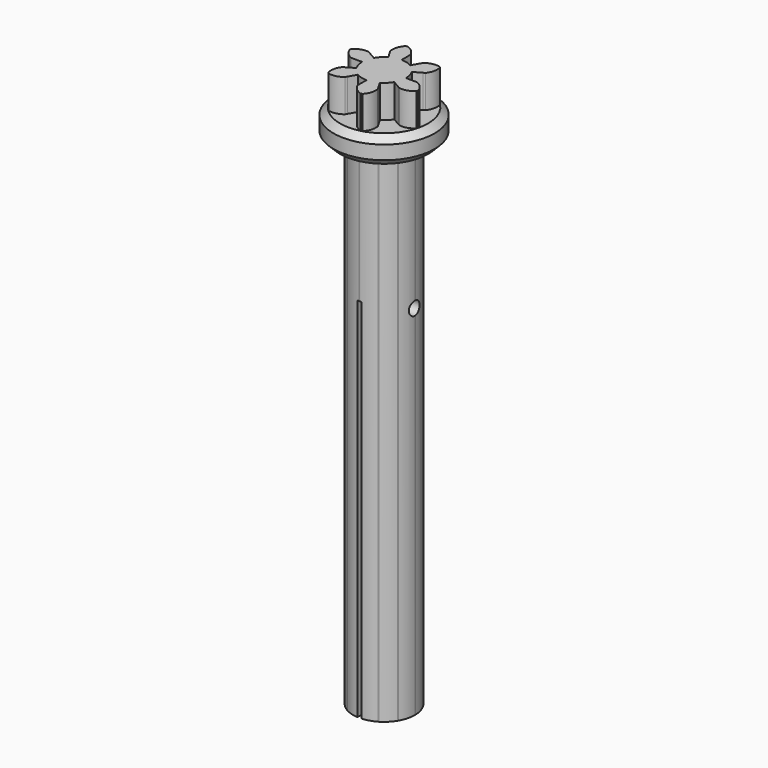
from build123d import *

# Parameters (mm, degrees)
F6_DEPTH       = 5
F7_DEPTH       = 80
F9_START       = -75.9
F8_R           = 7.6984631039
F9_DEPTH       = 4.1
F10_SIZE       = 1
F11_DEPTH      = 55.9
F12_R          = 1.025
F13_DEPTH      = 7.6994631039
F13_DEPTH_BACK = 7.6994631039


# Not quite as in the source:
# - a feature names something its author has since deleted; it is built from what else it names


with BuildPart() as f6:
    # F5 (on Top) → F6 (new body)
    with BuildSketch(Plane.XY):
        with BuildLine():
            Line((-4.0689884067, 2.349231552), (-4.3301270189, 2.5))
            ThreePointArc((-4.3301270189, 2.5), (-4.8296291314, 1.2940952255), (-5, 0))
            Line((-5, 0), (-4.6984631039, 0))
            ThreePointArc((-4.6984631039, 0), (-4.538366856, 1.216051734), (-4.0689884067, 2.349231552))
        make_face()
        with BuildLine():
            Line((-2.8867513459, 1.6666666667), (-4.0689884067, 2.349231552))
            ThreePointArc((-4.0689884067, 2.349231552), (-4.538366856, 1.216051734), (-4.6984631039, 0))
            Line((-4.6984631039, 0), (-3.3333333333, 0))
            ThreePointArc((-3.3333333333, 0), (-3.2197527543, 0.8627301503), (-2.8867513459, 1.6666666667))
        make_face()
        with BuildLine():
            ThreePointArc((-2.5, 4.3301270189), (-1.2940952255, 4.8296291314), (0, 5))
            ThreePointArc((0, 5), (-0.6289197853, 5.9186828799), (-1.5943250641, 6.4732196035))
            Line((-1.5943250641, 6.4732196035), (-1.7258162456, 6.440833913))
            Line((-1.7258162456, 6.440833913), (-1.8558837944, 6.4031351529))
            ThreePointArc((-1.8558837944, 6.4031351529), (-2.414680929, 5.4401896236), (-2.5, 4.3301270189))
        make_face()
        with BuildLine():
            ThreePointArc((2.8867513459, -1.6666666667), (3.2197527543, -0.8627301503), (3.3333333333, 0))
            ThreePointArc((3.3333333333, 0), (3.2197527543, 0.8627301503), (2.8867513459, 1.6666666667))
            ThreePointArc((2.8867513459, 1.6666666667), (2.357022604, 2.357022604), (1.6666666667, 2.8867513459))
            ThreePointArc((1.6666666667, 2.8867513459), (0.8627301503, 3.2197527543), (0, 3.3333333333))
            ThreePointArc((0, 3.3333333333), (-0.8627301503, 3.2197527543), (-1.6666666667, 2.8867513459))
            ThreePointArc((-1.6666666667, 2.8867513459), (-2.357022604, 2.357022604), (-2.8867513459, 1.6666666667))
            ThreePointArc((-2.8867513459, 1.6666666667), (-3.2197527543, 0.8627301503), (-3.3333333333, 0))
            ThreePointArc((-3.3333333333, 0), (-3.2197527543, -0.8627301503), (-2.8867513459, -1.6666666667))
            ThreePointArc((-2.8867513459, -1.6666666667), (-2.357022604, -2.357022604), (-1.6666666667, -2.8867513459))
            ThreePointArc((-1.6666666667, -2.8867513459), (-0.8627301503, -3.2197527543), (0, -3.3333333333))
            ThreePointArc((0, -3.3333333333), (0.8627301503, -3.2197527543), (1.6666666667, -2.8867513459))
            ThreePointArc((1.6666666667, -2.8867513459), (2.357022604, -2.357022604), (2.8867513459, -1.6666666667))
        make_face()
        with BuildLine():
            Line((4.0689884067, 2.349231552), (4.3301270189, 2.5))
            ThreePointArc((4.3301270189, 2.5), (3.5355339059, 3.5355339059), (2.5, 4.3301270189))
            Line((2.5, 4.3301270189), (2.349231552, 4.0689884067))
            ThreePointArc((2.349231552, 4.0689884067), (3.3223151219, 3.3223151219), (4.0689884067, 2.349231552))
        make_face()
        with BuildLine():
            Line((2.8867513459, 1.6666666667), (4.0689884067, 2.349231552))
            ThreePointArc((4.0689884067, 2.349231552), (3.3223151219, 3.3223151219), (2.349231552, 4.0689884067))
            Line((2.349231552, 4.0689884067), (1.6666666667, 2.8867513459))
            ThreePointArc((1.6666666667, 2.8867513459), (2.357022604, 2.357022604), (2.8867513459, 1.6666666667))
        make_face()
        with BuildLine():
            ThreePointArc((4.3301270189, -2.5), (4.8296291314, -1.2940952255), (5, 0))
            Line((5, 0), (4.6984631039, 0))
            ThreePointArc((4.6984631039, 0), (4.538366856, -1.216051734), (4.0689884067, -2.349231552))
            Line((4.0689884067, -2.349231552), (4.3301270189, -2.5))
        make_face()
        with BuildLine():
            ThreePointArc((4.0689884067, -2.349231552), (4.538366856, -1.216051734), (4.6984631039, 0))
            Line((4.6984631039, 0), (3.3333333333, 0))
            ThreePointArc((3.3333333333, 0), (3.2197527543, -0.8627301503), (2.8867513459, -1.6666666667))
            Line((2.8867513459, -1.6666666667), (4.0689884067, -2.349231552))
        make_face()
        with BuildLine():
            ThreePointArc((0, -5), (1.2940952255, -4.8296291314), (2.5, -4.3301270189))
            Line((2.5, -4.3301270189), (2.349231552, -4.0689884067))
            ThreePointArc((2.349231552, -4.0689884067), (1.216051734, -4.538366856), (0, -4.6984631039))
            Line((0, -4.6984631039), (0, -5))
        make_face()
        with BuildLine():
            ThreePointArc((0, -4.6984631039), (1.216051734, -4.538366856), (2.349231552, -4.0689884067))
            Line((2.349231552, -4.0689884067), (1.6666666667, -2.8867513459))
            ThreePointArc((1.6666666667, -2.8867513459), (0.8627301503, -3.2197527543), (0, -3.3333333333))
            Line((0, -3.3333333333), (0, -4.6984631039))
        make_face()
        with BuildLine():
            ThreePointArc((-4.3301270189, -2.5), (-3.5355339059, -3.5355339059), (-2.5, -4.3301270189))
            Line((-2.5, -4.3301270189), (-2.349231552, -4.0689884067))
            ThreePointArc((-2.349231552, -4.0689884067), (-3.3223151219, -3.3223151219), (-4.0689884067, -2.349231552))
            Line((-4.0689884067, -2.349231552), (-4.3301270189, -2.5))
        make_face()
        with BuildLine():
            ThreePointArc((-4.0689884067, -2.349231552), (-3.3223151219, -3.3223151219), (-2.349231552, -4.0689884067))
            Line((-2.349231552, -4.0689884067), (-1.6666666667, -2.8867513459))
            ThreePointArc((-1.6666666667, -2.8867513459), (-2.357022604, -2.357022604), (-2.8867513459, -1.6666666667))
            Line((-2.8867513459, -1.6666666667), (-4.0689884067, -2.349231552))
        make_face()
        with BuildLine():
            Line((0, 4.6984631039), (0, 5))
            ThreePointArc((0, 5), (-1.2940952255, 4.8296291314), (-2.5, 4.3301270189))
            Line((-2.5, 4.3301270189), (-2.349231552, 4.0689884067))
            ThreePointArc((-2.349231552, 4.0689884067), (-1.216051734, 4.538366856), (0, 4.6984631039))
        make_face()
        with BuildLine():
            Line((0, 3.3333333333), (0, 4.6984631039))
            ThreePointArc((0, 4.6984631039), (-1.216051734, 4.538366856), (-2.349231552, 4.0689884067))
            Line((-2.349231552, 4.0689884067), (-1.6666666667, 2.8867513459))
            ThreePointArc((-1.6666666667, 2.8867513459), (-0.8627301503, 3.2197527543), (0, 3.3333333333))
        make_face()
        with BuildLine():
            ThreePointArc((-5, 0), (-4.8296291314, 1.2940952255), (-4.3301270189, 2.5))
            ThreePointArc((-4.3301270189, 2.5), (-5.4401896236, 2.414680929), (-6.4031351529, 1.8558837944))
            Line((-6.4031351529, 1.8558837944), (-6.440833913, 1.7258162456))
            Line((-6.440833913, 1.7258162456), (-6.4732196035, 1.5943250641))
            ThreePointArc((-6.4732196035, 1.5943250641), (-5.9186828799, 0.6289197853), (-5, 0))
        make_face()
        with BuildLine():
            ThreePointArc((-4.6173358091, -4.8088100888), (-3.5040019509, -4.8112698383), (-2.5, -4.3301270189))
            ThreePointArc((-2.5, -4.3301270189), (-3.5355339059, -3.5355339059), (-4.3301270189, -2.5))
            ThreePointArc((-4.3301270189, -2.5), (-4.8112698383, -3.5040019509), (-4.8088100888, -4.6173358091))
            Line((-4.8088100888, -4.6173358091), (-4.7150176674, -4.7150176674))
            Line((-4.7150176674, -4.7150176674), (-4.6173358091, -4.8088100888))
        make_face()
        with BuildLine():
            ThreePointArc((1.8558837944, -6.4031351529), (2.414680929, -5.4401896236), (2.5, -4.3301270189))
            ThreePointArc((2.5, -4.3301270189), (1.2940952255, -4.8296291314), (0, -5))
            ThreePointArc((0, -5), (0.6289197853, -5.9186828799), (1.5943250641, -6.4732196035))
            Line((1.5943250641, -6.4732196035), (1.7258162456, -6.440833913))
            Line((1.7258162456, -6.440833913), (1.8558837944, -6.4031351529))
        make_face()
        with BuildLine():
            ThreePointArc((6.4732196035, -1.5943250641), (5.9186828799, -0.6289197853), (5, 0))
            ThreePointArc((5, 0), (4.8296291314, -1.2940952255), (4.3301270189, -2.5))
            ThreePointArc((4.3301270189, -2.5), (5.4401896236, -2.414680929), (6.4031351529, -1.8558837944))
            Line((6.4031351529, -1.8558837944), (6.440833913, -1.7258162456))
            Line((6.440833913, -1.7258162456), (6.4732196035, -1.5943250641))
        make_face()
        with BuildLine():
            ThreePointArc((2.5, 4.3301270189), (3.5355339059, 3.5355339059), (4.3301270189, 2.5))
            ThreePointArc((4.3301270189, 2.5), (4.8112698383, 3.5040019509), (4.8088100888, 4.6173358091))
            Line((4.8088100888, 4.6173358091), (4.7150176674, 4.7150176674))
            Line((4.7150176674, 4.7150176674), (4.6173358091, 4.8088100888))
            ThreePointArc((4.6173358091, 4.8088100888), (3.5040019509, 4.8112698383), (2.5, 4.3301270189))
        make_face()
    extrude(amount=F6_DEPTH)

    # F5 (on Top) → F7 (join)
    with BuildSketch(Plane.XY):
        with BuildLine():
            ThreePointArc((2.8867513459, -1.6666666667), (3.2197527543, -0.8627301503), (3.3333333333, 0))
            ThreePointArc((3.3333333333, 0), (3.2197527543, 0.8627301503), (2.8867513459, 1.6666666667))
            ThreePointArc((2.8867513459, 1.6666666667), (2.357022604, 2.357022604), (1.6666666667, 2.8867513459))
            ThreePointArc((1.6666666667, 2.8867513459), (0.8627301503, 3.2197527543), (0, 3.3333333333))
            ThreePointArc((0, 3.3333333333), (-0.8627301503, 3.2197527543), (-1.6666666667, 2.8867513459))
            ThreePointArc((-1.6666666667, 2.8867513459), (-2.357022604, 2.357022604), (-2.8867513459, 1.6666666667))
            ThreePointArc((-2.8867513459, 1.6666666667), (-3.2197527543, 0.8627301503), (-3.3333333333, 0))
            ThreePointArc((-3.3333333333, 0), (-3.2197527543, -0.8627301503), (-2.8867513459, -1.6666666667))
            ThreePointArc((-2.8867513459, -1.6666666667), (-2.357022604, -2.357022604), (-1.6666666667, -2.8867513459))
            ThreePointArc((-1.6666666667, -2.8867513459), (-0.8627301503, -3.2197527543), (0, -3.3333333333))
            ThreePointArc((0, -3.3333333333), (0.8627301503, -3.2197527543), (1.6666666667, -2.8867513459))
            ThreePointArc((1.6666666667, -2.8867513459), (2.357022604, -2.357022604), (2.8867513459, -1.6666666667))
        make_face()
        with BuildLine():
            ThreePointArc((-4.1169236265, -2.2641765374), (-4.0931769499, -2.306828558), (-4.0689884067, -2.349231552))
            Line((-4.0689884067, -2.349231552), (-2.8867513459, -1.6666666667))
            ThreePointArc((-2.8867513459, -1.6666666667), (-3.2197527543, -0.8627301503), (-3.3333333333, 0))
            Line((-3.3333333333, 0), (-4.6984631039, 0))
            ThreePointArc((-4.6984631039, 0), (-4.6982094998, -0.0488163415), (-4.6974487147, -0.0976274132))
            ThreePointArc((-4.6974487147, -0.0976274132), (-4.538366856, -1.216051734), (-4.1169236265, -2.2641765374))
        make_face()
        with BuildLine():
            Line((-2.8867513459, 1.6666666667), (-4.0689884067, 2.349231552))
            ThreePointArc((-4.0689884067, 2.349231552), (-4.538366856, 1.216051734), (-4.6984631039, 0))
            Line((-4.6984631039, 0), (-3.3333333333, 0))
            ThreePointArc((-3.3333333333, 0), (-3.2197527543, 0.8627301503), (-2.8867513459, 1.6666666667))
        make_face()
        with BuildLine():
            ThreePointArc((-2.349231552, 4.0689884067), (-2.3913809418, 4.0443606083), (-2.4332721773, 4.0192962133))
            ThreePointArc((-2.4332721773, 4.0192962133), (-3.3223151219, 3.3223151219), (-4.0192962133, 2.4332721773))
            ThreePointArc((-4.0192962133, 2.4332721773), (-4.0443606083, 2.3913809418), (-4.0689884067, 2.349231552))
            Line((-4.0689884067, 2.349231552), (-2.8867513459, 1.6666666667))
            ThreePointArc((-2.8867513459, 1.6666666667), (-2.357022604, 2.357022604), (-1.6666666667, 2.8867513459))
            Line((-1.6666666667, 2.8867513459), (-2.349231552, 4.0689884067))
        make_face()
        with BuildLine():
            Line((0, 3.3333333333), (0, 4.6984631039))
            ThreePointArc((0, 4.6984631039), (-1.216051734, 4.538366856), (-2.349231552, 4.0689884067))
            Line((-2.349231552, 4.0689884067), (-1.6666666667, 2.8867513459))
            ThreePointArc((-1.6666666667, 2.8867513459), (-0.8627301503, 3.2197527543), (0, 3.3333333333))
        make_face()
        with BuildLine():
            ThreePointArc((2.349231552, 4.0689884067), (2.306828558, 4.0931769499), (2.2641765374, 4.1169236265))
            ThreePointArc((2.2641765374, 4.1169236265), (1.216051734, 4.538366856), (0.0976274132, 4.6974487147))
            ThreePointArc((0.0976274132, 4.6974487147), (0.0488163415, 4.6982094998), (0, 4.6984631039))
            Line((0, 4.6984631039), (0, 3.3333333333))
            ThreePointArc((0, 3.3333333333), (0.8627301503, 3.2197527543), (1.6666666667, 2.8867513459))
            Line((1.6666666667, 2.8867513459), (2.349231552, 4.0689884067))
        make_face()
        with BuildLine():
            Line((2.8867513459, 1.6666666667), (4.0689884067, 2.349231552))
            ThreePointArc((4.0689884067, 2.349231552), (3.3223151219, 3.3223151219), (2.349231552, 4.0689884067))
            Line((2.349231552, 4.0689884067), (1.6666666667, 2.8867513459))
            ThreePointArc((1.6666666667, 2.8867513459), (2.357022604, 2.357022604), (2.8867513459, 1.6666666667))
        make_face()
        with BuildLine():
            ThreePointArc((4.6984631039, 0), (4.6982094998, 0.0488163415), (4.6974487147, 0.0976274132))
            ThreePointArc((4.6974487147, 0.0976274132), (4.538366856, 1.216051734), (4.1169236265, 2.2641765374))
            ThreePointArc((4.1169236265, 2.2641765374), (4.0931769499, 2.306828558), (4.0689884067, 2.349231552))
            Line((4.0689884067, 2.349231552), (2.8867513459, 1.6666666667))
            ThreePointArc((2.8867513459, 1.6666666667), (3.2197527543, 0.8627301503), (3.3333333333, 0))
            Line((3.3333333333, 0), (4.6984631039, 0))
        make_face()
        with BuildLine():
            ThreePointArc((4.0689884067, -2.349231552), (4.538366856, -1.216051734), (4.6984631039, 0))
            Line((4.6984631039, 0), (3.3333333333, 0))
            ThreePointArc((3.3333333333, 0), (3.2197527543, -0.8627301503), (2.8867513459, -1.6666666667))
            Line((2.8867513459, -1.6666666667), (4.0689884067, -2.349231552))
        make_face()
        with BuildLine():
            ThreePointArc((4.0192962133, -2.4332721773), (4.0443606083, -2.3913809418), (4.0689884067, -2.349231552))
            Line((4.0689884067, -2.349231552), (2.8867513459, -1.6666666667))
            ThreePointArc((2.8867513459, -1.6666666667), (2.357022604, -2.357022604), (1.6666666667, -2.8867513459))
            Line((1.6666666667, -2.8867513459), (2.349231552, -4.0689884067))
            ThreePointArc((2.349231552, -4.0689884067), (2.3913809418, -4.0443606083), (2.4332721773, -4.0192962133))
            ThreePointArc((2.4332721773, -4.0192962133), (3.3223151219, -3.3223151219), (4.0192962133, -2.4332721773))
        make_face()
        with BuildLine():
            ThreePointArc((0, -4.6984631039), (1.216051734, -4.538366856), (2.349231552, -4.0689884067))
            Line((2.349231552, -4.0689884067), (1.6666666667, -2.8867513459))
            ThreePointArc((1.6666666667, -2.8867513459), (0.8627301503, -3.2197527543), (0, -3.3333333333))
            Line((0, -3.3333333333), (0, -4.6984631039))
        make_face()
        with BuildLine():
            ThreePointArc((-0.0976274132, -4.6974487147), (-0.0488163415, -4.6982094998), (0, -4.6984631039))
            Line((0, -4.6984631039), (0, -3.3333333333))
            ThreePointArc((0, -3.3333333333), (-0.8627301503, -3.2197527543), (-1.6666666667, -2.8867513459))
            Line((-1.6666666667, -2.8867513459), (-2.349231552, -4.0689884067))
            ThreePointArc((-2.349231552, -4.0689884067), (-2.306828558, -4.0931769499), (-2.2641765374, -4.1169236265))
            ThreePointArc((-2.2641765374, -4.1169236265), (-1.216051734, -4.538366856), (-0.0976274132, -4.6974487147))
        make_face()
        with BuildLine():
            ThreePointArc((-4.0689884067, -2.349231552), (-3.3223151219, -3.3223151219), (-2.349231552, -4.0689884067))
            Line((-2.349231552, -4.0689884067), (-1.6666666667, -2.8867513459))
            ThreePointArc((-1.6666666667, -2.8867513459), (-2.357022604, -2.357022604), (-2.8867513459, -1.6666666667))
            Line((-2.8867513459, -1.6666666667), (-4.0689884067, -2.349231552))
        make_face()
    extrude(amount=-F7_DEPTH)

    # F8 (on face) → F9 (join)
    with BuildSketch(Plane(origin=(0, 0, -80), x_dir=(1, 0, 0), z_dir=(0, 0, -1)).offset(F9_START)):
        Circle(F8_R)
        with BuildLine():
            ThreePointArc((-0.3, -4.6888757223), (-4.6984631039, 0), (-0.3, 4.6888757223))
            ThreePointArc((-0.3, 4.6888757223), (0, 4.6984631039), (0.3, 4.6888757223))
            ThreePointArc((0.3, 4.6888757223), (3.4267400303, 3.2144996973), (4.6984631039, 0))
            ThreePointArc((4.6984631039, 0), (3.4267400303, -3.2144996973), (0.3, -4.6888757223))
            ThreePointArc((0.3, -4.6888757223), (0, -4.6984631039), (-0.3, -4.6888757223))
        make_face(mode=Mode.SUBTRACT)
    extrude(amount=-F9_DEPTH)

    # F10
    f10_edges = [f6.edges().sort_by_distance(p)[0] for p in [
        (-7.698463, 0, 0),
        (-7.698463, 0, -4.1),
    ]]
    chamfer(f10_edges, length=F10_SIZE)

    # F8 (on face) → F11 (cut)
    with BuildSketch(Plane(origin=(0, 0, -80), x_dir=(1, 0, 0), z_dir=(0, 0, -1))):
        with BuildLine():
            ThreePointArc((0.3, 4.6888757223), (0, 4.6984631039), (-0.3, 4.6888757223))
            Line((-0.3, 4.6888757223), (-0.3, -4.6888757223))
            ThreePointArc((-0.3, -4.6888757223), (0, -4.6984631039), (0.3, -4.6888757223))
            Line((0.3, -4.6888757223), (0.3, 4.6888757223))
        make_face()
    extrude(amount=-F11_DEPTH, mode=Mode.SUBTRACT)

    # F12 (on Right) → F13 (cut, two sides)
    with BuildSketch(Plane.YZ) as f13_sk:
        with Locations((0, -25.425)):
            Circle(F12_R)
    extrude(amount=F13_DEPTH, mode=Mode.SUBTRACT)
    extrude(f13_sk.sketch, amount=-F13_DEPTH_BACK, mode=Mode.SUBTRACT)


solid = f6.part
